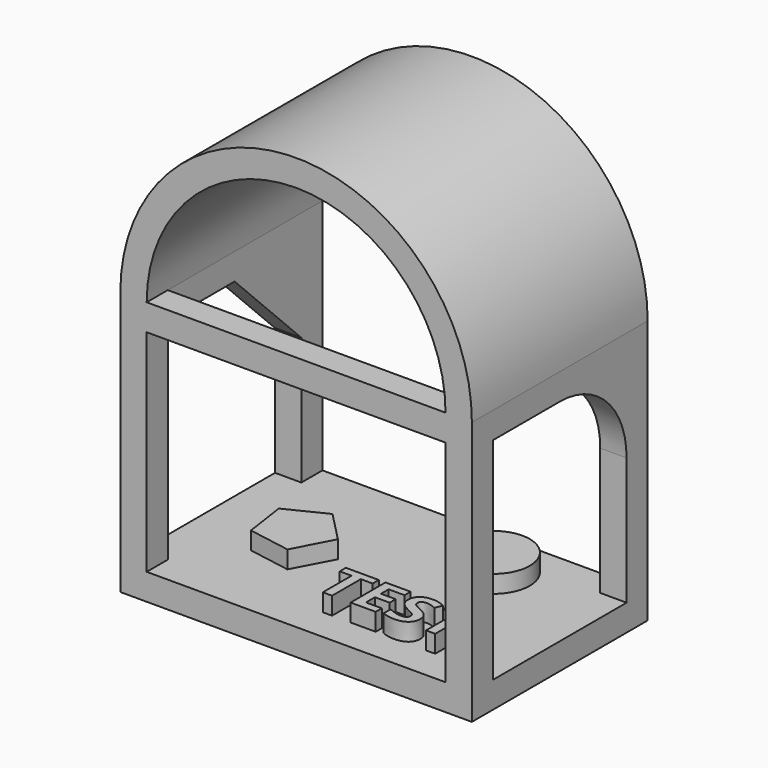
from build123d import *

# Parameters (mm, degrees)
F1_DEPTH     = 25
F2_W         = 19
F2_H         = 24
F3_DEPTH     = 40.001
F4_SIZE      = 9.5
F5_R         = 9.5
F6_W         = 3
F6_H         = 3
F7_DEPTH     = 37
F8_R         = 4.1375135908
F8_TEXT_SIZE = 6.943113274
F9_DEPTH     = 2


# Not quite as in the source:
# - Text() gives the source's letters only with a copy of the font that has no kerning and outlines rounded to 1/6400 em; it was checked with that copy


with BuildPart() as f1:
    # F0 (on Front) → F1 (new body)
    with BuildSketch(Plane.XZ):
        with BuildLine():
            Line((-20, -15), (20, -15))
            Line((20, -15), (20, 15))
            ThreePointArc((20, 15), (0, 35), (-20, 15))
            Line((-20, 15), (-20, -15))
        make_face()
        with BuildLine():
            ThreePointArc((-17, 15), (0, 32), (17, 15))
            Line((17, 15), (17, -12))
            Line((17, -12), (-17, -12))
            Line((-17, -12), (-17, 15))
        make_face(mode=Mode.SUBTRACT)
    extrude(amount=F1_DEPTH)

    # F2 (on face) → F3 (cut, through all)
    with BuildSketch(Plane.YZ.offset(20)):
        with Locations((-12.5, 0)):
            Rectangle(F2_W, F2_H)
    extrude(amount=-F3_DEPTH, mode=Mode.SUBTRACT)

    # F4
    f4_edges = [f1.edges().sort_by_distance(p)[0] for p in [
        (-18.5, -3, 12),
    ]]
    chamfer(f4_edges, length=F4_SIZE)

    # F5
    f5_edges = [f1.edges().sort_by_distance(p)[0] for p in [
        (18.5, -3, 12),
    ]]
    fillet(f5_edges, radius=F5_R)

    # F6 (on face) → F7 (join, through all)
    with BuildSketch(Plane.YZ.offset(20)):
        with Locations((-23.5, 13.5)):
            Rectangle(F6_W, F6_H)
    extrude(amount=-F7_DEPTH)

    # F8 (on face) → F9 (join)
    with BuildSketch(Plane.XY.offset(-12)):
        Polygon((-5.2510312507, -12.495173729), (-8.6621633982, -8.9945843155), (-13.0455195743, -11.1570221532), (-12.3434505286, -15.9940716489), (-7.5261918197, -16.8210948048), align=None)
        with Locations((7.1177319624, -5.8399410918)):
            Circle(F8_R)
        with Locations((-1.4064222341, -21.2964713573)):
            Text('TEST', F8_TEXT_SIZE, font='Open Sans', font_style=FontStyle.BOLD, text_align=(TextAlign.LEFT, TextAlign.BOTTOM))
    extrude(amount=F9_DEPTH)


solid = f1.part
